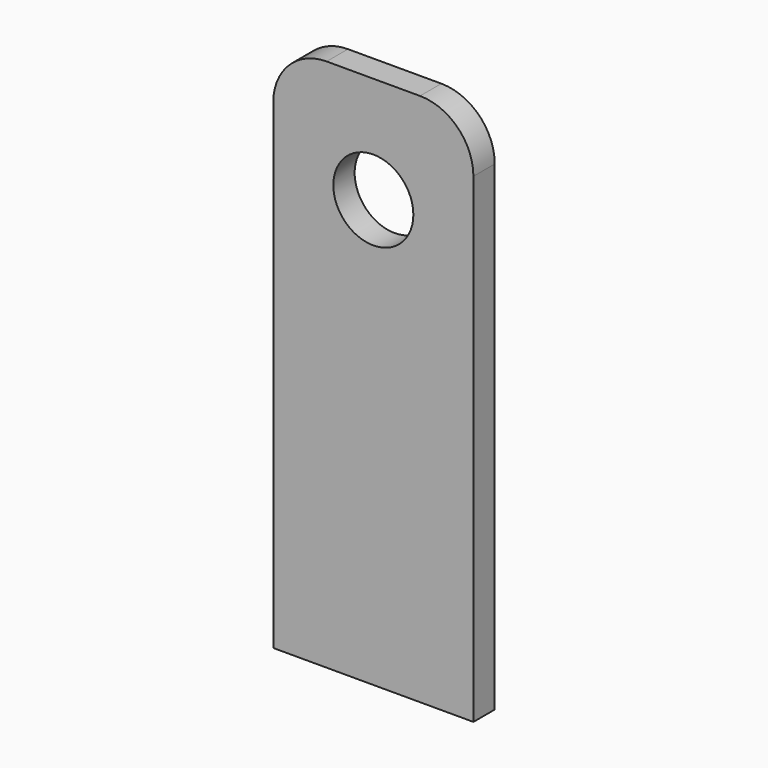
from build123d import *

# Parameters (mm, degrees)
F0_W          = 75
F0_H          = 200
F1_DEPTH      = 10
F2_R          = 15
F3_DEPTH      = 219
F3_DEPTH_BACK = 25
F4_R          = 20


# Not quite as in the source:
# - an extrude ends at something that could not be found from the text; its depth is read off the source's solid


with BuildPart() as f1:
    # F0 (on Front) → F1 (new body)
    with BuildSketch(Plane.XZ):
        Rectangle(F0_W, F0_H)
    extrude(amount=F1_DEPTH)

    # F2 (on Front) → F3 (cut, two sides)
    with BuildSketch(Plane.XZ) as f3_sk:
        with Locations((0, 60)):
            Circle(F2_R)
    extrude(amount=-F3_DEPTH, mode=Mode.SUBTRACT)
    extrude(f3_sk.sketch, amount=F3_DEPTH_BACK, mode=Mode.SUBTRACT)

    # F4
    f4_edges = [f1.edges().sort_by_distance(p)[0] for p in [
        (-37.5, -5, 100),
        (37.5, -5, 100),
    ]]
    fillet(f4_edges, radius=F4_R)


solid = f1.part
